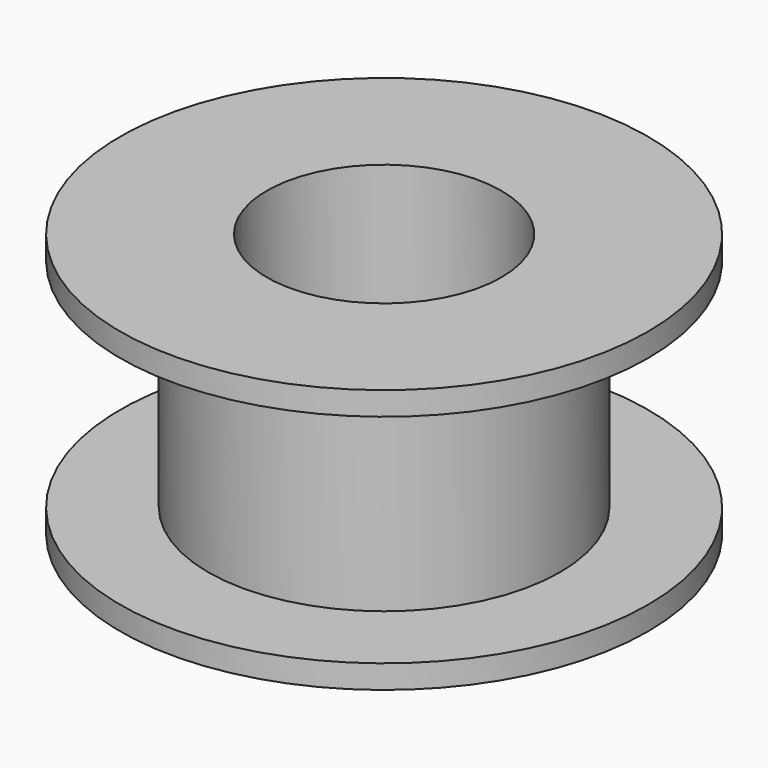
from build123d import *

# Parameters (mm, degrees)
F0_R     = 6
F1_DEPTH = 7.4
F2_R     = 9
F3_DEPTH = 0.8
F4_R     = 9
F5_DEPTH = 0.8
F6_R     = 4
F7_DEPTH = 9.001


# Not quite as in the source:
# - ends of sketch curves that miss each other by under 0.0002 mm in the source are joined


with BuildPart() as f1:
    # F0 (on Top) → F1 (new body)
    with BuildSketch(Plane.XY):
        Circle(F0_R)
        with BuildLine():
            ThreePointArc((0.3806045388, -5.7658808945), (0.3821052842, -5.7646171302), (0.3836035472, -5.7633504238))
            ThreePointArc((0.3836035472, -5.7633504238), (0, -5.25), (-0.3836035472, -5.7633504238))
            ThreePointArc((-0.3836035472, -5.7633504238), (-0.3821052842, -5.7646171302), (-0.3806045388, -5.7658808945))
            ThreePointArc((-0.3806045388, -5.7658808945), (-0.3463448965, -5.8591249109), (-0.4093829562, -5.9358997292))
            ThreePointArc((-0.4093829562, -5.9358997292), (-0.4525361238, -5.9421469593), (-0.4942455569, -5.9294368476))
            ThreePointArc((-0.4942455569, -5.9294368476), (-0.9311233557, -5.8766920369), (-1.3629081057, -5.7918029572))
            ThreePointArc((-1.3629081057, -5.7918029572), (-1.4044855806, -5.7906197903), (-1.441985055, -5.7726232426))
            ThreePointArc((-1.441985055, -5.7726232426), (-1.4799897199, -5.6798690996), (-1.4184467175, -5.6007480248))
            ThreePointArc((-1.4184467175, -5.6007480248), (-1.4166288992, -5.6000098693), (-1.4148125327, -5.5992681488))
            ThreePointArc((-1.4148125327, -5.5992681488), (-1.6210071809, -4.9925028678), (-2.1444698391, -5.3621881184))
            ThreePointArc((-2.1444698391, -5.3621881184), (-2.1434363401, -5.3638558164), (-2.1423995711, -5.3655214836))
            ThreePointArc((-2.1423995711, -5.3655214836), (-2.1392066719, -5.4658737363), (-2.2247634424, -5.5184171304))
            ThreePointArc((-2.2247634424, -5.5184171304), (-2.2652635999, -5.5109390447), (-2.2993151455, -5.4877727597))
            ThreePointArc((-2.2993151455, -5.4877727597), (-2.7009268548, -5.3016501323), (-3.0875904018, -5.0861857527))
            ThreePointArc((-3.0875904018, -5.0861857527), (-3.1238007071, -5.0726605298), (-3.1521764439, -5.0464129504))
            ThreePointArc((-3.1521764439, -5.0464129504), (-3.1620439351, -4.945353315), (-3.078417275, -4.8877599211))
            ThreePointArc((-3.078417275, -4.8877599211), (-3.0764603245, -4.8876196303), (-3.0745036529, -4.8874755002))
            ThreePointArc((-3.0745036529, -4.8874755002), (-3.0831056333, -4.2466897755), (-3.6951872305, -4.4365224847))
            ThreePointArc((-3.6951872305, -4.4365224847), (-3.6947196616, -4.4384279285), (-3.6942483551, -4.4403324513))
            ThreePointArc((-3.6942483551, -4.4403324513), (-3.7234373447, -4.5379012507), (-3.8230076712, -4.5592885789))
            ThreePointArc((-3.8230076712, -4.5592885789), (-3.8560268582, -4.5406730269), (-3.8797455624, -4.5111056706))
            ThreePointArc((-3.8797455624, -4.5111056706), (-4.2068112489, -4.2077593938), (-4.5102312248, -3.8807620771))
            ThreePointArc((-4.5102312248, -3.8807620771), (-4.5371123267, -3.8585413389), (-4.5547275545, -3.8284405316))
            ThreePointArc((-4.5547275545, -3.8284405316), (-4.535446501, -3.7270635192), (-4.4368176497, -3.6967088266))
            ThreePointArc((-4.4368176497, -3.6967088266), (-4.4349131269, -3.6971801331), (-4.433007683, -3.697647702))
            ThreePointArc((-4.433007683, -3.697647702), (-4.2431749738, -3.0855661048), (-4.8839606986, -3.0769641244))
            ThreePointArc((-4.8839606986, -3.0769641244), (-4.8841048286, -3.0789207959), (-4.8842451195, -3.0808777465))
            ThreePointArc((-4.8842451195, -3.0808777465), (-4.9440169669, -3.1654857116), (-5.0466911586, -3.1517310085))
            ThreePointArc((-5.0466911586, -3.1517310085), (-5.069110444, -3.1263184325), (-5.0817550004, -3.0948773992))
            ThreePointArc((-5.0817550004, -3.0948773992), (-5.3012375926, -2.7017364763), (-5.4903626511, -2.2931240611))
            ThreePointArc((-5.4903626511, -2.2931240611), (-5.5060730233, -2.2671022941), (-5.5132397924, -2.2375627347))
            ThreePointArc((-5.5132397924, -2.2375627347), (-5.4658096238, -2.1437373386), (-5.3606781484, -2.144183121))
            ThreePointArc((-5.3606781484, -2.144183121), (-5.3590124813, -2.14521989), (-5.3573447832, -2.146253389))
            ThreePointArc((-5.3573447832, -2.146253389), (-4.9876595327, -1.6227907307), (-5.5944248136, -1.4165960825))
            ThreePointArc((-5.5944248136, -1.4165960825), (-5.5951665342, -1.4184124491), (-5.5959046897, -1.4202302674))
            ThreePointArc((-5.5959046897, -1.4202302674), (-5.6812065984, -1.4824247971), (-5.7747415985, -1.4334781025))
            ThreePointArc((-5.7747415985, -1.4334781025), (-5.7857648681, -1.4063168524), (-5.7884387811, -1.3771261661))
            ThreePointArc((-5.7884387811, -1.3771261661), (-5.8767455172, -0.9307857571), (-5.9306876982, -0.4790025331))
            ThreePointArc((-5.9306876982, -0.4790025331), (-5.8853739929, -0.3594639118), (-5.7595648686, -0.3821548374))
            ThreePointArc((-5.7595648686, -0.3821548374), (-5.7583011043, -0.3836555828), (-5.7570343979, -0.3851538458))
            ThreePointArc((-5.7570343979, -0.3851538458), (-5.2436839741, -0.0015502986), (-5.7570343979, 0.3820532486))
            ThreePointArc((-5.7570343979, 0.3820532486), (-5.7583011043, 0.3805549856), (-5.7595648686, 0.3790542403))
            ThreePointArc((-5.7595648686, 0.3790542403), (-5.8622942172, 0.3468784197), (-5.9346909264, 0.426548483))
            ThreePointArc((-5.9346909264, 0.426548483), (-5.9358323151, 0.4509676612), (-5.9310148859, 0.4749341254))
            ThreePointArc((-5.9310148859, 0.4749341254), (-5.8765991635, 0.9317093277), (-5.7870583583, 1.3829156003))
            ThreePointArc((-5.7870583583, 1.3829156003), (-5.7843038364, 1.4029349854), (-5.7775807433, 1.4219918266))
            ThreePointArc((-5.7775807433, 1.4219918266), (-5.6843404021, 1.4793255219), (-5.594431999, 1.416896419))
            ThreePointArc((-5.594431999, 1.416896419), (-5.5936938435, 1.4150786007), (-5.5929521229, 1.4132622341))
            ThreePointArc((-5.5929521229, 1.4132622341), (-4.986186842, 1.6194568823), (-5.3558720925, 2.1429195405))
            ThreePointArc((-5.3558720925, 2.1429195405), (-5.3575397905, 2.1418860415), (-5.3592054577, 2.1408492726))
            ThreePointArc((-5.3592054577, 2.1408492726), (-5.4688284086, 2.1433207754), (-5.5102834557, 2.2448332315))
            ThreePointArc((-5.5102834557, 2.2448332315), (-5.5046167329, 2.2637285902), (-5.4953509969, 2.2811438842))
            ThreePointArc((-5.4953509969, 2.2811438842), (-5.3005253653, 2.7031335247), (-5.0733549953, 3.1086281688))
            ThreePointArc((-5.0733549953, 3.1086281688), (-5.0663266491, 3.1222793914), (-5.0572912917, 3.1346937317))
            ThreePointArc((-5.0572912917, 3.1346937317), (-4.9499559959, 3.164809758), (-4.8814438952, 3.0768669764))
            ThreePointArc((-4.8814438952, 3.0768669764), (-4.8813036044, 3.0749100259), (-4.8811594743, 3.0729533544))
            ThreePointArc((-4.8811594743, 3.0729533544), (-4.2403737496, 3.0815553348), (-4.4302064588, 3.6936369319))
            ThreePointArc((-4.4302064588, 3.6936369319), (-4.4321119026, 3.693169363), (-4.4340164255, 3.6926980566))
            ThreePointArc((-4.4340164255, 3.6926980566), (-4.538656044, 3.7304491107), (-4.5436525599, 3.841577985))
            ThreePointArc((-4.5436525599, 3.841577985), (-4.5343248359, 3.8545144167), (-4.523059132, 3.8658034209))
            ThreePointArc((-4.523059132, 3.8658034209), (-4.2049856642, 4.2095837756), (-3.8608578947, 4.5272813384))
            ThreePointArc((-3.8608578947, 4.5272813384), (-3.852175731, 4.5356041669), (-3.8425571832, 4.5428244841))
            ThreePointArc((-3.8425571832, 4.5428244841), (-3.729720065, 4.5410442426), (-3.6903928007, 4.4352673511))
            ThreePointArc((-3.6903928007, 4.4352673511), (-3.6908641072, 4.4333628283), (-3.6913316761, 4.4314573845))
            ThreePointArc((-3.6913316761, 4.4314573845), (-3.0792500789, 4.2416246753), (-3.0706480985, 4.8824104))
            ThreePointArc((-3.0706480985, 4.8824104), (-3.0726047701, 4.8825545301), (-3.0745617206, 4.8826948209))
            ThreePointArc((-3.0745617206, 4.8826948209), (-3.1626644803, 4.9516976688), (-3.1315994665, 5.0592079204))
            ThreePointArc((-3.1315994665, 5.0592079204), (-3.119936027, 5.0676010486), (-3.1071900735, 5.074235888))
            ThreePointArc((-3.1071900735, 5.074235888), (-2.6977366196, 5.3032741897), (-2.2715103211, 5.4993400387))
            ThreePointArc((-2.2715103211, 5.4993400387), (-2.1503267928, 5.4810489954), (-2.1378670951, 5.3591278498))
            ThreePointArc((-2.1378670951, 5.3591278498), (-2.1389038641, 5.3574621827), (-2.1399373631, 5.3557944847))
            ThreePointArc((-2.1399373631, 5.3557944847), (-1.6164747048, 4.9861092341), (-1.4102800566, 5.592874515))
            ThreePointArc((-1.4102800566, 5.592874515), (-1.4120964232, 5.5936162356), (-1.4139142415, 5.5943543911))
            ThreePointArc((-1.4139142415, 5.5943543911), (-1.4763804938, 5.6864908439), (-1.4149370546, 5.7793125137))
            ThreePointArc((-1.4149370546, 5.7793125137), (-1.3999049739, 5.7842378178), (-1.3842842971, 5.7867311139))
            ThreePointArc((-1.3842842971, 5.7867311139), (-0.9264014664, 5.8774382449), (-0.4628171036, 5.9319727181))
            ThreePointArc((-0.4628171036, 5.9319727181), (-0.4476995944, 5.9342860016), (-0.4324061315, 5.9342670093))
            ThreePointArc((-0.4324061315, 5.9342670093), (-0.3449604214, 5.8651285474), (-0.3758388115, 5.7580145701))
            ThreePointArc((-0.3758388115, 5.7580145701), (-0.3773395569, 5.7567508057), (-0.3788378199, 5.7554840994))
            ThreePointArc((-0.3788378199, 5.7554840994), (0.0047657273, 5.2421336756), (0.3883692745, 5.7554840994))
            ThreePointArc((0.3883692745, 5.7554840994), (0.3868710115, 5.7567508057), (0.3853702662, 5.7580145701))
            ThreePointArc((0.3853702662, 5.7580145701), (0.3538873578, 5.8631766757), (0.4378708106, 5.9338662905))
            ThreePointArc((0.4378708106, 5.9338662905), (0.4573929959, 5.9342736516), (0.4766221718, 5.9308794715))
            ThreePointArc((0.4766221718, 5.9308794715), (0.9358457669, 5.8759418565), (1.3894149145, 5.785501378))
            ThreePointArc((1.3894149145, 5.785501378), (1.4093589983, 5.7827272829), (1.4283429976, 5.7760138748))
            ThreePointArc((1.4283429976, 5.7760138748), (1.4856410056, 5.6827706834), (1.4232124448, 5.5928817004))
            ThreePointArc((1.4232124448, 5.5928817004), (1.4213946265, 5.5921435449), (1.41957826, 5.5914018243))
            ThreePointArc((1.41957826, 5.5914018243), (1.6257729082, 4.9846365434), (2.1492355664, 5.3543217939))
            ThreePointArc((2.1492355664, 5.3543217939), (2.1482020674, 5.355989492), (2.1471652984, 5.3576551591))
            ThreePointArc((2.1471652984, 5.3576551591), (2.1484055829, 5.4654463163), (2.2467992931, 5.5094820933))
            ThreePointArc((2.2467992931, 5.5094820933), (2.2701462131, 5.5030245881), (2.2912554418, 5.4911427318))
            ThreePointArc((2.2912554418, 5.4911427318), (2.7064393495, 5.298838179), (3.1056182667, 5.0751980436))
            ThreePointArc((3.1056182667, 5.0751980436), (3.1286854235, 5.0647208158), (3.1483792489, 5.048782834))
            ThreePointArc((3.1483792489, 5.048782834), (3.169420639, 4.9436317748), (3.0831830023, 4.8798935967))
            ThreePointArc((3.0831830023, 4.8798935967), (3.0812260518, 4.8797533058), (3.0792693802, 4.8796091758))
            ThreePointArc((3.0792693802, 4.8796091758), (3.0878713606, 4.238823451), (3.6999529578, 4.4286561602))
            ThreePointArc((3.6999529578, 4.4286561602), (3.6994853889, 4.4305616041), (3.6990140824, 4.4324661269))
            ThreePointArc((3.6990140824, 4.4324661269), (3.7316088821, 4.5330409603), (3.8362478957, 4.5481537004))
            ThreePointArc((3.8362478957, 4.5481537004), (3.8609061096, 4.53271015), (3.8800750956, 4.5108222369))
            ThreePointArc((3.8800750956, 4.5108222369), (4.2117676312, 4.2027982846), (4.5190837616, 3.8704498389))
            ThreePointArc((4.5190837616, 3.8704498389), (4.5419784366, 3.8505567927), (4.5578563234, 3.8247151182))
            ThreePointArc((4.5578563234, 3.8247151182), (4.5416785998, 3.7208726241), (4.441583377, 3.6888425022))
            ThreePointArc((4.441583377, 3.6888425022), (4.4396788542, 3.6893138086), (4.4377734103, 3.6897813775))
            ThreePointArc((4.4377734103, 3.6897813775), (4.2479407012, 3.0776997804), (4.8887264259, 3.0690978))
            ThreePointArc((4.8887264259, 3.0690978), (4.8888705559, 3.0710544715), (4.8890108468, 3.073011422))
            ThreePointArc((4.8890108468, 3.073011422), (4.9489466875, 3.1576907408), (5.0517351443, 3.1436399335))
            ThreePointArc((5.0517351443, 3.1436399335), (5.0739585149, 3.1183183587), (5.0865115484, 3.0870536549))
            ThreePointArc((5.0865115484, 3.0870536549), (5.3044458004, 2.6954322011), (5.4922842876, 2.2885177089))
            ThreePointArc((5.4922842876, 2.2885177089), (5.5108977286, 2.2590924146), (5.5182939971, 2.2250688442))
            ThreePointArc((5.5182939971, 2.2250688442), (5.4685840303, 2.1346836809), (5.3654438757, 2.1363167965))
            ThreePointArc((5.3654438757, 2.1363167965), (5.3637782086, 2.1373535655), (5.3621105105, 2.1383870645))
            ThreePointArc((5.3621105105, 2.1383870645), (4.99242526, 1.6149244063), (5.5991905409, 1.4087297581))
            ThreePointArc((5.5991905409, 1.4087297581), (5.5999322615, 1.4105461246), (5.600670417, 1.4123639429))
            ThreePointArc((5.600670417, 1.4123639429), (5.6817933965, 1.4741605567), (5.7749452179, 1.4326575759))
            ThreePointArc((5.7749452179, 1.4326575759), (5.7905658496, 1.3983050131), (5.7923433498, 1.3606096128))
            ThreePointArc((5.7923433498, 1.3606096128), (5.8777300273, 0.9245483905), (5.9303365162, 0.4833309479))
            ThreePointArc((5.9303365162, 0.4833309479), (5.9406046173, 0.4461148884), (5.9360098784, 0.407782691))
            ThreePointArc((5.9360098784, 0.407782691), (5.8600341125, 0.3404768743), (5.7643305959, 0.374288513))
            ThreePointArc((5.7643305959, 0.374288513), (5.7630668316, 0.3757892583), (5.7618001253, 0.3772875213))
            ThreePointArc((5.7618001253, 0.3772875213), (5.2484497014, -0.0063160259), (5.7618001253, -0.3899195731))
            ThreePointArc((5.7618001253, -0.3899195731), (5.7630668316, -0.3884213101), (5.7643305959, -0.3869205647))
            ThreePointArc((5.7643305959, -0.3869205647), (5.8589130817, -0.352896847), (5.9352813712, -0.4182523696))
            ThreePointArc((5.9352813712, -0.4182523696), (5.9405882849, -0.4589613406), (5.9290914374, -0.4983720771))
            ThreePointArc((5.9290914374, -0.4983720771), (5.8758462536, -0.9364458362), (5.7902789498, -1.3693683519))
            ThreePointArc((5.7902789498, -1.3693683519), (5.7890432658, -1.4109094735), (5.7710268611, -1.4483607867))
            ThreePointArc((5.7710268611, -1.4483607867), (5.6782814399, -1.4863006219), (5.5991977263, -1.4247627434))
            ThreePointArc((5.5991977263, -1.4247627434), (5.5984595708, -1.4229449251), (5.5977178502, -1.4211285585))
            ThreePointArc((5.5977178502, -1.4211285585), (4.9909525693, -1.6273232067), (5.3606378198, -2.150785865))
            ThreePointArc((5.3606378198, -2.150785865), (5.3623055179, -2.149752366), (5.363971185, -2.148715597))
            ThreePointArc((5.363971185, -2.148715597), (5.4965423161, -2.1730904294), (5.4844051341, -2.3073361968))
            ThreePointArc((5.4844051341, -2.3073361968), (5.2993121671, -2.705511145), (5.0853590441, -3.0889518275))
            ThreePointArc((5.0853590441, -3.0889518275), (5.0710792206, -3.130167057), (5.0406318988, -3.1614126685))
            ThreePointArc((5.0406318988, -3.1614126685), (4.9414861677, -3.167246403), (4.8862096226, -3.0847333009))
            ThreePointArc((4.8862096226, -3.0847333009), (4.8860693317, -3.0827763503), (4.8859252016, -3.0808196788))
            ThreePointArc((4.8859252016, -3.0808196788), (4.2451394769, -3.0894216592), (4.4349721861, -3.7015032564))
            ThreePointArc((4.4349721861, -3.7015032564), (4.43687763, -3.7010356874), (4.4387821528, -3.700564381))
            ThreePointArc((4.4387821528, -3.700564381), (4.5338661391, -3.7271588755), (4.5597701404, -3.8224332913))
            ThreePointArc((4.5597701404, -3.8224332913), (4.2049311669, -4.2096382127), (3.8173294995, -4.5640437653))
            ThreePointArc((3.8173294995, -4.5640437653), (3.7218637964, -4.5383274637), (3.695158528, -4.4431336756))
            ThreePointArc((3.695158528, -4.4431336756), (3.6956298345, -4.4412291528), (3.6960974034, -4.4393237089))
            ThreePointArc((3.6960974034, -4.4393237089), (3.0840158062, -4.2494909997), (3.0754138259, -4.8902767244))
            ThreePointArc((3.0754138259, -4.8902767244), (3.0773704974, -4.8904208545), (3.0793274479, -4.8905611454))
            ThreePointArc((3.0793274479, -4.8905611454), (3.1614118111, -4.944984516), (3.1570355374, -5.0433745266))
            ThreePointArc((3.1570355374, -5.0433745266), (2.6997840023, -5.3022322036), (2.2214782118, -5.5197404427))
            ThreePointArc((2.2214782118, -5.5197404427), (2.1386184867, -5.4657888682), (2.1426328224, -5.3669941743))
            ThreePointArc((2.1426328224, -5.3669941743), (2.1436695914, -5.3653285072), (2.1447030904, -5.3636608091))
            ThreePointArc((2.1447030904, -5.3636608091), (1.6212404321, -4.9939755586), (1.4150457839, -5.6007408395))
            ThreePointArc((1.4150457839, -5.6007408395), (1.4168621505, -5.6014825601), (1.4186799688, -5.6022207156))
            ThreePointArc((1.4186799688, -5.6022207156), (1.4799653708, -5.6795779085), (1.4450020565, -5.7718687664))
            ThreePointArc((1.4450020565, -5.7718687664), (0.9728192286, -5.8699337942), (0.4942455569, -5.9294368476))
            ThreePointArc((0.4942455569, -5.9294368476), (0.4525361238, -5.9421469593), (0.4093829562, -5.9358997292))
            ThreePointArc((0.4093829562, -5.9358997292), (0.3463448965, -5.8591249109), (0.3806045388, -5.7658808945))
        make_face(mode=Mode.SUBTRACT)
        with BuildLine():
            ThreePointArc((-0.3836035472, -5.7633504238), (0, -5.25), (0.3836035472, -5.7633504238))
            ThreePointArc((0.3836035472, -5.7633504238), (0.3821052842, -5.7646171302), (0.3806045388, -5.7658808945))
            ThreePointArc((0.3806045388, -5.7658808945), (0.3463448965, -5.8591249109), (0.4093829562, -5.9358997292))
            ThreePointArc((0.4093829562, -5.9358997292), (0.4518258123, -5.9328200238), (0.4942455569, -5.9294368476))
            ThreePointArc((0.4942455569, -5.9294368476), (0.9728192286, -5.8699337942), (1.4450020565, -5.7718687664))
            ThreePointArc((1.4450020565, -5.7718687664), (1.4799653708, -5.6795779085), (1.4186799688, -5.6022207156))
            ThreePointArc((1.4186799688, -5.6022207156), (1.4168621505, -5.6014825601), (1.4150457839, -5.6007408395))
            ThreePointArc((1.4150457839, -5.6007408395), (1.6212404321, -4.9939755586), (2.1447030904, -5.3636608091))
            ThreePointArc((2.1447030904, -5.3636608091), (2.1436695914, -5.3653285072), (2.1426328224, -5.3669941743))
            ThreePointArc((2.1426328224, -5.3669941743), (2.1386184867, -5.4657888682), (2.2214782118, -5.5197404427))
            ThreePointArc((2.2214782118, -5.5197404427), (2.6997840023, -5.3022322036), (3.1570355374, -5.0433745266))
            ThreePointArc((3.1570355374, -5.0433745266), (3.1614118111, -4.944984516), (3.0793274479, -4.8905611454))
            ThreePointArc((3.0793274479, -4.8905611454), (3.0773704974, -4.8904208545), (3.0754138259, -4.8902767244))
            ThreePointArc((3.0754138259, -4.8902767244), (3.0840158062, -4.2494909997), (3.6960974034, -4.4393237089))
            ThreePointArc((3.6960974034, -4.4393237089), (3.6956298345, -4.4412291528), (3.695158528, -4.4431336756))
            ThreePointArc((3.695158528, -4.4431336756), (3.7218637964, -4.5383274637), (3.8173294995, -4.5640437653))
            ThreePointArc((3.8173294995, -4.5640437653), (4.2049311669, -4.2096382127), (4.5597701404, -3.8224332913))
            ThreePointArc((4.5597701404, -3.8224332913), (4.5338661391, -3.7271588755), (4.4387821528, -3.700564381))
            ThreePointArc((4.4387821528, -3.700564381), (4.43687763, -3.7010356874), (4.4349721861, -3.7015032564))
            ThreePointArc((4.4349721861, -3.7015032564), (4.2451394769, -3.0894216592), (4.8859252016, -3.0808196788))
            ThreePointArc((4.8859252016, -3.0808196788), (4.8860693317, -3.0827763503), (4.8862096226, -3.0847333009))
            ThreePointArc((4.8862096226, -3.0847333009), (4.9414861677, -3.167246403), (5.0406318988, -3.1614126685))
            ThreePointArc((5.0406318988, -3.1614126685), (5.0631251009, -3.125262263), (5.0853590441, -3.0889518275))
            ThreePointArc((5.0853590441, -3.0889518275), (5.2993121671, -2.705511145), (5.4844051341, -2.3073361968))
            ThreePointArc((5.4844051341, -2.3073361968), (5.4965423161, -2.1730904294), (5.363971185, -2.148715597))
            ThreePointArc((5.363971185, -2.148715597), (5.3623055179, -2.149752366), (5.3606378198, -2.150785865))
            ThreePointArc((5.3606378198, -2.150785865), (4.9909525693, -1.6273232067), (5.5977178502, -1.4211285585))
            ThreePointArc((5.5977178502, -1.4211285585), (5.5984595708, -1.4229449251), (5.5991977263, -1.4247627434))
            ThreePointArc((5.5991977263, -1.4247627434), (5.6782814399, -1.4863006219), (5.7710268611, -1.4483607867))
            ThreePointArc((5.7710268611, -1.4483607867), (5.7807878325, -1.4088974538), (5.7902789498, -1.3693683519))
            ThreePointArc((5.7902789498, -1.3693683519), (5.8758462536, -0.9364458362), (5.9290914374, -0.4983720771))
            ThreePointArc((5.9290914374, -0.4983720771), (5.9323216642, -0.4583226733), (5.9352813712, -0.4182523696))
            ThreePointArc((5.9352813712, -0.4182523696), (5.8589130817, -0.352896847), (5.7643305959, -0.3869205647))
            ThreePointArc((5.7643305959, -0.3869205647), (5.7630668316, -0.3884213101), (5.7618001253, -0.3899195731))
            ThreePointArc((5.7618001253, -0.3899195731), (5.2484497014, -0.0063160259), (5.7618001253, 0.3772875213))
            ThreePointArc((5.7618001253, 0.3772875213), (5.7630668316, 0.3757892583), (5.7643305959, 0.374288513))
            ThreePointArc((5.7643305959, 0.374288513), (5.8600341125, 0.3404768743), (5.9360098784, 0.407782691))
            ThreePointArc((5.9360098784, 0.407782691), (5.9332934424, 0.4455658494), (5.9303365162, 0.4833309479))
            ThreePointArc((5.9303365162, 0.4833309479), (5.8777300273, 0.9245483905), (5.7923433498, 1.3606096128))
            ThreePointArc((5.7923433498, 1.3606096128), (5.7837564722, 1.3966606856), (5.7749452179, 1.4326575759))
            ThreePointArc((5.7749452179, 1.4326575759), (5.6817933965, 1.4741605567), (5.600670417, 1.4123639429))
            ThreePointArc((5.600670417, 1.4123639429), (5.5999322615, 1.4105461246), (5.5991905409, 1.4087297581))
            ThreePointArc((5.5991905409, 1.4087297581), (4.99242526, 1.6149244063), (5.3621105105, 2.1383870645))
            ThreePointArc((5.3621105105, 2.1383870645), (5.3637782086, 2.1373535655), (5.3654438757, 2.1363167965))
            ThreePointArc((5.3654438757, 2.1363167965), (5.4685840303, 2.1346836809), (5.5182939971, 2.2250688442))
            ThreePointArc((5.5182939971, 2.2250688442), (5.5053805482, 2.2568307467), (5.4922842876, 2.2885177089))
            ThreePointArc((5.4922842876, 2.2885177089), (5.3044458004, 2.6954322011), (5.0865115484, 3.0870536549))
            ThreePointArc((5.0865115484, 3.0870536549), (5.0692023043, 3.1153953197), (5.0517351443, 3.1436399335))
            ThreePointArc((5.0517351443, 3.1436399335), (4.9489466875, 3.1576907408), (4.8890108468, 3.073011422))
            ThreePointArc((4.8890108468, 3.073011422), (4.8888705559, 3.0710544715), (4.8887264259, 3.0690978))
            ThreePointArc((4.8887264259, 3.0690978), (4.2479407012, 3.0776997804), (4.4377734103, 3.6897813775))
            ThreePointArc((4.4377734103, 3.6897813775), (4.4396788542, 3.6893138086), (4.441583377, 3.6888425022))
            ThreePointArc((4.441583377, 3.6888425022), (4.5416785998, 3.7208726241), (4.5578563234, 3.8247151182))
            ThreePointArc((4.5578563234, 3.8247151182), (4.5385276514, 3.8476313177), (4.5190837616, 3.8704498389))
            ThreePointArc((4.5190837616, 3.8704498389), (4.2117676312, 4.2027982846), (3.8800750956, 4.5108222369))
            ThreePointArc((3.8800750956, 4.5108222369), (3.8582066477, 4.5295409772), (3.8362478957, 4.5481537004))
            ThreePointArc((3.8362478957, 4.5481537004), (3.7316088821, 4.5330409603), (3.6990140824, 4.4324661269))
            ThreePointArc((3.6990140824, 4.4324661269), (3.6994853889, 4.4305616041), (3.6999529578, 4.4286561602))
            ThreePointArc((3.6999529578, 4.4286561602), (3.0878713606, 4.238823451), (3.0792693802, 4.8796091758))
            ThreePointArc((3.0792693802, 4.8796091758), (3.0812260518, 4.8797533058), (3.0831830023, 4.8798935967))
            ThreePointArc((3.0831830023, 4.8798935967), (3.169420639, 4.9436317748), (3.1483792489, 5.048782834))
            ThreePointArc((3.1483792489, 5.048782834), (3.1270266504, 5.0620355913), (3.1056182667, 5.0751980436))
            ThreePointArc((3.1056182667, 5.0751980436), (2.7064393495, 5.298838179), (2.2912554418, 5.4911427318))
            ThreePointArc((2.2912554418, 5.4911427318), (2.2690458958, 5.5003573268), (2.2467992931, 5.5094820933))
            ThreePointArc((2.2467992931, 5.5094820933), (2.1484055829, 5.4654463163), (2.1471652984, 5.3576551591))
            ThreePointArc((2.1471652984, 5.3576551591), (2.1482020674, 5.355989492), (2.1492355664, 5.3543217939))
            ThreePointArc((2.1492355664, 5.3543217939), (1.6257729082, 4.9846365434), (1.41957826, 5.5914018243))
            ThreePointArc((1.41957826, 5.5914018243), (1.4213946265, 5.5921435449), (1.4232124448, 5.5928817004))
            ThreePointArc((1.4232124448, 5.5928817004), (1.4856410056, 5.6827706834), (1.4283429976, 5.7760138748))
            ThreePointArc((1.4283429976, 5.7760138748), (1.4088869422, 5.7807903944), (1.3894149145, 5.785501378))
            ThreePointArc((1.3894149145, 5.785501378), (0.9358457669, 5.8759418565), (0.4766221718, 5.9308794715))
            ThreePointArc((0.4766221718, 5.9308794715), (0.45724893, 5.9324045223), (0.4378708106, 5.9338662905))
            ThreePointArc((0.4378708106, 5.9338662905), (0.3538873578, 5.8631766757), (0.3853702662, 5.7580145701))
            ThreePointArc((0.3853702662, 5.7580145701), (0.3868710115, 5.7567508057), (0.3883692745, 5.7554840994))
            ThreePointArc((0.3883692745, 5.7554840994), (0.0047657273, 5.2421336756), (-0.3788378199, 5.7554840994))
            ThreePointArc((-0.3788378199, 5.7554840994), (-0.3773395569, 5.7567508057), (-0.3758388115, 5.7580145701))
            ThreePointArc((-0.3758388115, 5.7580145701), (-0.3449604214, 5.8651285474), (-0.4324061315, 5.9342670093))
            ThreePointArc((-0.4324061315, 5.9342670093), (-0.4476130875, 5.9331393481), (-0.4628171036, 5.9319727181))
            ThreePointArc((-0.4628171036, 5.9319727181), (-0.9264014664, 5.8774382449), (-1.3842842971, 5.7867311139))
            ThreePointArc((-1.3842842971, 5.7867311139), (-1.3996155911, 5.7830421231), (-1.4149370546, 5.7793125137))
            ThreePointArc((-1.4149370546, 5.7793125137), (-1.4763804938, 5.6864908439), (-1.4139142415, 5.5943543911))
            ThreePointArc((-1.4139142415, 5.5943543911), (-1.4120964232, 5.5936162356), (-1.4102800566, 5.592874515))
            ThreePointArc((-1.4102800566, 5.592874515), (-1.6164747048, 4.9861092341), (-2.1399373631, 5.3557944847))
            ThreePointArc((-2.1399373631, 5.3557944847), (-2.1389038641, 5.3574621827), (-2.1378670951, 5.3591278498))
            ThreePointArc((-2.1378670951, 5.3591278498), (-2.1503267928, 5.4810489954), (-2.2715103211, 5.4993400387))
            ThreePointArc((-2.2715103211, 5.4993400387), (-2.6977366196, 5.3032741897), (-3.1071900735, 5.074235888))
            ThreePointArc((-3.1071900735, 5.074235888), (-3.1194038198, 5.0667366035), (-3.1315994665, 5.0592079204))
            ThreePointArc((-3.1315994665, 5.0592079204), (-3.1626644803, 4.9516976688), (-3.0745617206, 4.8826948209))
            ThreePointArc((-3.0745617206, 4.8826948209), (-3.0726047701, 4.8825545301), (-3.0706480985, 4.8824104))
            ThreePointArc((-3.0706480985, 4.8824104), (-3.0792500789, 4.2416246753), (-3.6913316761, 4.4314573845))
            ThreePointArc((-3.6913316761, 4.4314573845), (-3.6908641072, 4.4333628283), (-3.6903928007, 4.4352673511))
            ThreePointArc((-3.6903928007, 4.4352673511), (-3.729720065, 4.5410442426), (-3.8425571832, 4.5428244841))
            ThreePointArc((-3.8425571832, 4.5428244841), (-3.8517153793, 4.5350621426), (-3.8608578947, 4.5272813384))
            ThreePointArc((-3.8608578947, 4.5272813384), (-4.2049856642, 4.2095837756), (-4.523059132, 3.8658034209))
            ThreePointArc((-4.523059132, 3.8658034209), (-4.533372028, 3.8537044588), (-4.5436525599, 3.841577985))
            ThreePointArc((-4.5436525599, 3.841577985), (-4.538656044, 3.7304491107), (-4.4340164255, 3.6926980566))
            ThreePointArc((-4.4340164255, 3.6926980566), (-4.4321119026, 3.693169363), (-4.4302064588, 3.6936369319))
            ThreePointArc((-4.4302064588, 3.6936369319), (-4.2403737496, 3.0815553348), (-4.8811594743, 3.0729533544))
            ThreePointArc((-4.8811594743, 3.0729533544), (-4.8813036044, 3.0749100259), (-4.8814438952, 3.0768669764))
            ThreePointArc((-4.8814438952, 3.0768669764), (-4.9499559959, 3.164809758), (-5.0572912917, 3.1346937317))
            ThreePointArc((-5.0572912917, 3.1346937317), (-5.0653399097, 3.121671283), (-5.0733549953, 3.1086281688))
            ThreePointArc((-5.0733549953, 3.1086281688), (-5.3005253653, 2.7031335247), (-5.4953509969, 2.2811438842))
            ThreePointArc((-5.4953509969, 2.2811438842), (-5.502847176, 2.2630008744), (-5.5102834557, 2.2448332315))
            ThreePointArc((-5.5102834557, 2.2448332315), (-5.4688284086, 2.1433207754), (-5.3592054577, 2.1408492726))
            ThreePointArc((-5.3592054577, 2.1408492726), (-5.3575397905, 2.1418860415), (-5.3558720925, 2.1429195405))
            ThreePointArc((-5.3558720925, 2.1429195405), (-4.986186842, 1.6194568823), (-5.5929521229, 1.4132622341))
            ThreePointArc((-5.5929521229, 1.4132622341), (-5.5936938435, 1.4150786007), (-5.594431999, 1.416896419))
            ThreePointArc((-5.594431999, 1.416896419), (-5.6843404021, 1.4793255219), (-5.7775807433, 1.4219918266))
            ThreePointArc((-5.7775807433, 1.4219918266), (-5.7823525598, 1.4024617195), (-5.7870583583, 1.3829156003))
            ThreePointArc((-5.7870583583, 1.3829156003), (-5.8765991635, 0.9317093277), (-5.9310148859, 0.4749341254))
            ThreePointArc((-5.9310148859, 0.4749341254), (-5.9329022323, 0.4507450517), (-5.9346909264, 0.426548483))
            ThreePointArc((-5.9346909264, 0.426548483), (-5.8622942172, 0.3468784197), (-5.7595648686, 0.3790542403))
            ThreePointArc((-5.7595648686, 0.3790542403), (-5.7583011043, 0.3805549856), (-5.7570343979, 0.3820532486))
            ThreePointArc((-5.7570343979, 0.3820532486), (-5.2436839741, -0.0015502986), (-5.7570343979, -0.3851538458))
            ThreePointArc((-5.7570343979, -0.3851538458), (-5.7583011043, -0.3836555828), (-5.7595648686, -0.3821548374))
            ThreePointArc((-5.7595648686, -0.3821548374), (-5.8853739929, -0.3594639118), (-5.9306876982, -0.4790025331))
            ThreePointArc((-5.9306876982, -0.4790025331), (-5.8767455172, -0.9307857571), (-5.7884387811, -1.3771261661))
            ThreePointArc((-5.7884387811, -1.3771261661), (-5.7816588457, -1.4053188221), (-5.7747415985, -1.4334781025))
            ThreePointArc((-5.7747415985, -1.4334781025), (-5.6812065984, -1.4824247971), (-5.5959046897, -1.4202302674))
            ThreePointArc((-5.5959046897, -1.4202302674), (-5.5951665342, -1.4184124491), (-5.5944248136, -1.4165960825))
            ThreePointArc((-5.5944248136, -1.4165960825), (-4.9876595327, -1.6227907307), (-5.3573447832, -2.146253389))
            ThreePointArc((-5.3573447832, -2.146253389), (-5.3590124813, -2.14521989), (-5.3606781484, -2.144183121))
            ThreePointArc((-5.3606781484, -2.144183121), (-5.4658096238, -2.1437373386), (-5.5132397924, -2.2375627347))
            ThreePointArc((-5.5132397924, -2.2375627347), (-5.5018713588, -2.2653722765), (-5.4903626511, -2.2931240611))
            ThreePointArc((-5.4903626511, -2.2931240611), (-5.3012375926, -2.7017364763), (-5.0817550004, -3.0948773992))
            ThreePointArc((-5.0817550004, -3.0948773992), (-5.0643028624, -3.1233534091), (-5.0466911586, -3.1517310085))
            ThreePointArc((-5.0466911586, -3.1517310085), (-4.9440169669, -3.1654857116), (-4.8842451195, -3.0808777465))
            ThreePointArc((-4.8842451195, -3.0808777465), (-4.8841048286, -3.0789207959), (-4.8839606986, -3.0769641244))
            ThreePointArc((-4.8839606986, -3.0769641244), (-4.2431749738, -3.0855661048), (-4.433007683, -3.697647702))
            ThreePointArc((-4.433007683, -3.697647702), (-4.4349131269, -3.6971801331), (-4.4368176497, -3.6967088266))
            ThreePointArc((-4.4368176497, -3.6967088266), (-4.535446501, -3.7270635192), (-4.5547275545, -3.8284405316))
            ThreePointArc((-4.5547275545, -3.8284405316), (-4.532554887, -3.8546655103), (-4.5102312248, -3.8807620771))
            ThreePointArc((-4.5102312248, -3.8807620771), (-4.2068112489, -4.2077593938), (-3.8797455624, -4.5111056706))
            ThreePointArc((-3.8797455624, -4.5111056706), (-3.8514519655, -4.5352858518), (-3.8230076712, -4.5592885789))
            ThreePointArc((-3.8230076712, -4.5592885789), (-3.7234373447, -4.5379012507), (-3.6942483551, -4.4403324513))
            ThreePointArc((-3.6942483551, -4.4403324513), (-3.6947196616, -4.4384279285), (-3.6951872305, -4.4365224847))
            ThreePointArc((-3.6951872305, -4.4365224847), (-3.0831056333, -4.2466897755), (-3.0745036529, -4.8874755002))
            ThreePointArc((-3.0745036529, -4.8874755002), (-3.0764603245, -4.8876196303), (-3.078417275, -4.8877599211))
            ThreePointArc((-3.078417275, -4.8877599211), (-3.1620439351, -4.945353315), (-3.1521764439, -5.0464129504))
            ThreePointArc((-3.1521764439, -5.0464129504), (-3.119946801, -5.0664022697), (-3.0875904018, -5.0861857527))
            ThreePointArc((-3.0875904018, -5.0861857527), (-2.7009268548, -5.3016501323), (-2.2993151455, -5.4877727597))
            ThreePointArc((-2.2993151455, -5.4877727597), (-2.2620911867, -5.5032211897), (-2.2247634424, -5.5184171304))
            ThreePointArc((-2.2247634424, -5.5184171304), (-2.1392066719, -5.4658737363), (-2.1423995711, -5.3655214836))
            ThreePointArc((-2.1423995711, -5.3655214836), (-2.1434363401, -5.3638558164), (-2.1444698391, -5.3621881184))
            ThreePointArc((-2.1444698391, -5.3621881184), (-1.6210071809, -4.9925028678), (-1.4148125327, -5.5992681488))
            ThreePointArc((-1.4148125327, -5.5992681488), (-1.4166288992, -5.6000098693), (-1.4184467175, -5.6007480248))
            ThreePointArc((-1.4184467175, -5.6007480248), (-1.4799897199, -5.6798690996), (-1.441985055, -5.7726232426))
            ThreePointArc((-1.441985055, -5.7726232426), (-1.4024793674, -5.7823482794), (-1.3629081057, -5.7918029572))
            ThreePointArc((-1.3629081057, -5.7918029572), (-0.9311233557, -5.8766920369), (-0.4942455569, -5.9294368476))
            ThreePointArc((-0.4942455569, -5.9294368476), (-0.4518258123, -5.9328200238), (-0.4093829562, -5.9358997292))
            ThreePointArc((-0.4093829562, -5.9358997292), (-0.3463448965, -5.8591249109), (-0.3806045388, -5.7658808945))
            ThreePointArc((-0.3806045388, -5.7658808945), (-0.3821052842, -5.7646171302), (-0.3836035472, -5.7633504238))
        make_face()
    extrude(amount=F1_DEPTH)

    # F2 (on face) → F3 (join)
    with BuildSketch(Plane.XY.offset(7.4)):
        Circle(F2_R)
    extrude(amount=F3_DEPTH)

    # F4 (on face) → F5 (join)
    with BuildSketch(Plane(origin=(0, 0, 0), x_dir=(1, 0, 0), z_dir=(0, 0, -1))):
        Circle(F4_R)
    extrude(amount=F5_DEPTH)

    # F6 (on face) → F7 (cut, through all)
    with BuildSketch(Plane(origin=(0, 0, -0.8), x_dir=(1, 0, 0), z_dir=(0, 0, -1))):
        Circle(F6_R)
    extrude(amount=-F7_DEPTH, mode=Mode.SUBTRACT)


solid = f1.part
